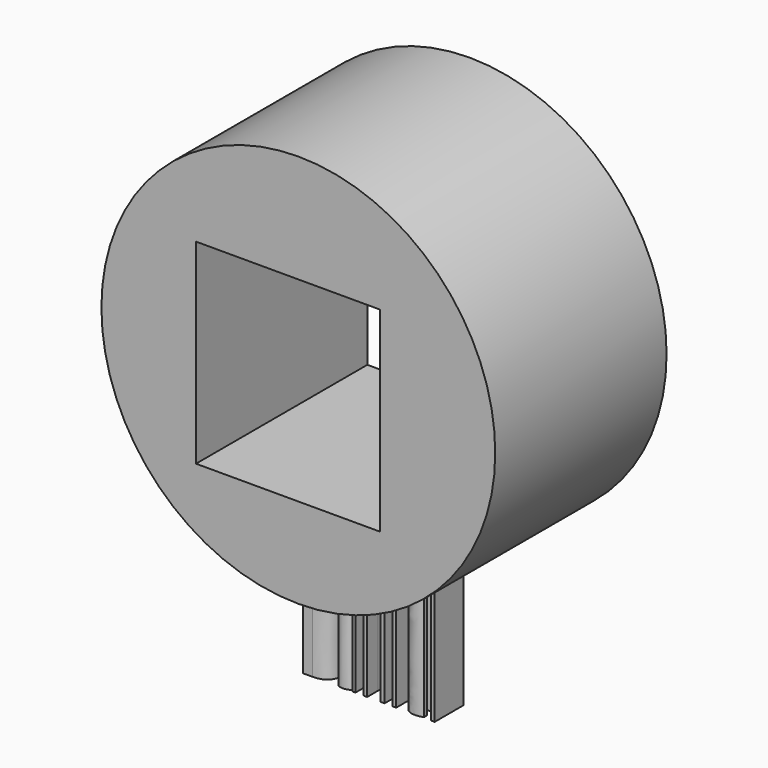
from build123d import *

# Parameters (mm, degrees)
F0_R         = 23.3517992909
F1_DEPTH     = 25.4
F2_W         = 21.8065371737
F2_H         = 23.1844373047
F3_DEPTH     = 25.4
F4_TEXT_SIZE = 5.6059073864
F5_DEPTH     = 25.4


# Not quite as in the source:
# - Text() gives the source's letters only with a copy of the font that has no kerning and outlines rounded to 1/6400 em; it was checked with that copy


with BuildPart() as f1:
    # F0 (on Front) → F1 (new body)
    with BuildSketch(Plane.XZ):
        Circle(F0_R)
    extrude(amount=F1_DEPTH)

    # F2 (on face) → F3 (cut)
    with BuildSketch(Plane.XZ.offset(25.4)):
        with Locations((-1.2300298549, -1.075591892)):
            Rectangle(F2_W, F2_H)
    extrude(amount=-F3_DEPTH, mode=Mode.SUBTRACT)

    # F4 (on face) → F5 (join)
    with BuildSketch(Plane.XY.offset(-12.6678105444)):
        with Locations((-9.1521427967, -13.9333084226)):
            Text('Daniel', F4_TEXT_SIZE, font='Open Sans', text_align=(TextAlign.LEFT, TextAlign.BOTTOM))
    extrude(amount=-F5_DEPTH)


solid = f1.part
